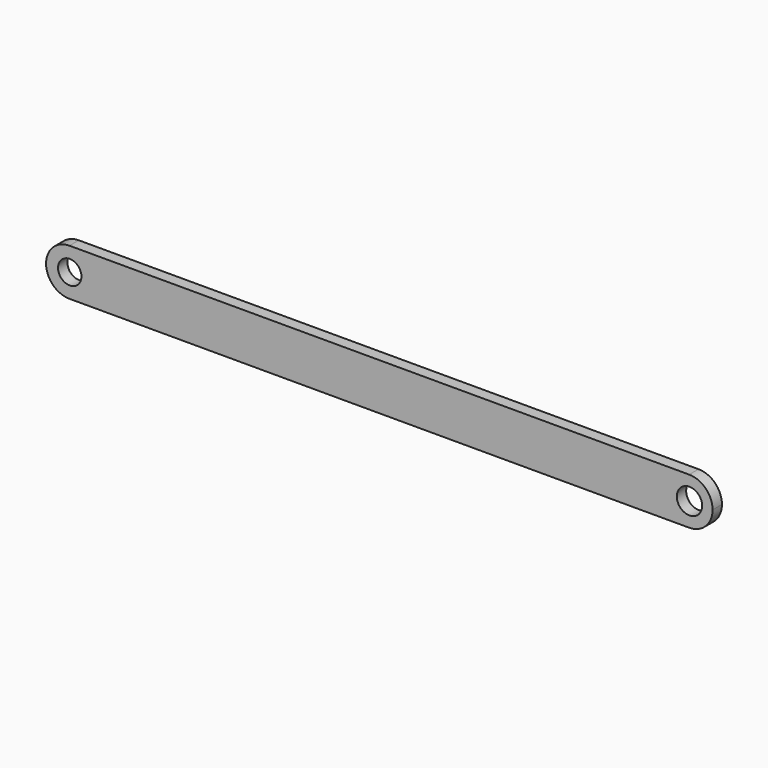
from build123d import *

# Parameters (mm, degrees)
F0_W     = 285
F0_H     = 20
F1_DEPTH = 5
F2_R     = 9.99999
F3_R     = 5
F3_R_2   = 5.4133078472
F4_DEPTH = 20


# Not quite as in the source:
# - a fillet or chamfer is up to 0.001 mm smaller than in the source, because OpenCascade refuses the exact size


with BuildPart() as f1:
    # F0 (on Front) → F1 (new body)
    with BuildSketch(Plane.XZ):
        with Locations((-142.5, 10)):
            Rectangle(F0_W, F0_H)
    extrude(amount=F1_DEPTH)

    # F2 (radius 10 in the source; OpenCascade refuses exactly that, so slightly less here)
    f2_edges = [f1.edges().sort_by_distance(p)[0] for p in [
        (0, -2.5, 20),
        (0, -2.5, 0),
        (-285, -2.5, 20),
        (-285, -2.5, 0),
    ]]
    fillet(f2_edges, radius=F2_R)

    # F3 (on Front) → F4 (cut)
    with BuildSketch(Plane.XZ):
        with Locations((-274.8824357986, 10.0639369339)):
            Circle(F3_R)
        with Locations((-9.8824357986, 10.070726499)):
            Circle(F3_R_2)
    extrude(amount=F4_DEPTH, mode=Mode.SUBTRACT)


solid = f1.part
